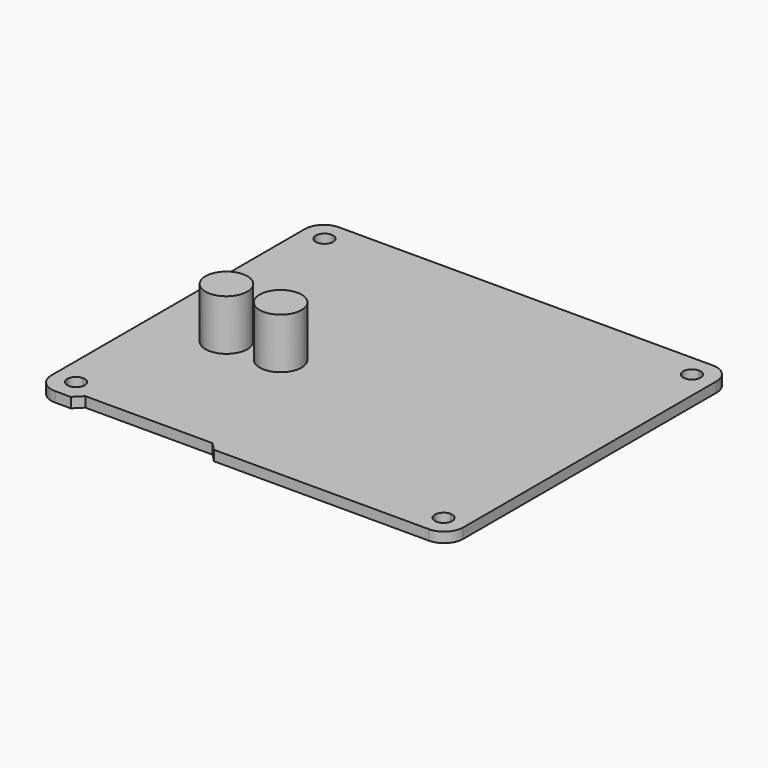
from build123d import *

# Parameters (mm, degrees)
F1_DEPTH = 1.6
F2_R     = 3.3061205596
F2_R_2   = 3.3042251001
F3_DEPTH = 8


# Not quite as in the source:
# - ends of sketch curves that miss each other by under 0.0002 mm in the source are joined


with BuildPart() as f1:
    # F0 (on Top) → F1 (new body)
    with BuildSketch(Plane.XY):
        with BuildLine():
            Line((-30.10027, 26.72715), (-30.10027, -23.27275))
            ThreePointArc((-30.10027, -23.27275), (-29.2216664958, -25.3938864958), (-27.10053, -26.27249))
            Line((-27.10053, -26.27249), (-24.63927, -26.27249))
            Line((-24.63927, -26.27249), (-23.36927, -25.00249))
            Line((-23.36927, -25.00249), (-3.30327, -25.00249))
            Line((-3.30327, -25.00249), (-2.03327, -26.27249))
            Line((-2.03327, -26.27249), (31.89859, -26.27249))
            ThreePointArc((31.89859, -26.27249), (34.020096129, -25.3935121782), (34.9008668601, -23.2727499955))
            Line((34.9008668601, -23.2727499955), (34.90087, 26.72715))
            ThreePointArc((34.90087, 26.72715), (34.0213682803, 28.8491843311), (31.8985900009, 29.7268889246))
            Line((31.8985900009, 29.7268889246), (-27.10053, 29.72689))
            ThreePointArc((-27.10053, 29.72689), (-29.2216664958, 28.8482864958), (-30.10027, 26.72715))
        make_face()
        with BuildLine():
            ThreePointArc((-26.60015, -24.14651), (-27.5718137123, -23.7440337123), (-27.97429, -22.77237))
            ThreePointArc((-27.97429, -22.77237), (-27.5718137123, -21.8007062877), (-26.60015, -21.39823))
            ThreePointArc((-26.60015, -21.39823), (-25.6284862877, -21.8007062877), (-25.22601, -22.77237))
            ThreePointArc((-25.22601, -22.77237), (-25.6284862877, -23.7440337123), (-26.60015, -24.14651))
        make_face(mode=Mode.SUBTRACT)
        with BuildLine():
            ThreePointArc((31.40075, -24.14651), (30.4290862877, -23.7440337123), (30.02661, -22.77237))
            ThreePointArc((30.02661, -22.77237), (30.4290862877, -21.8007062877), (31.40075, -21.39823))
            ThreePointArc((31.40075, -21.39823), (32.3724137123, -21.8007062877), (32.77489, -22.77237))
            ThreePointArc((32.77489, -22.77237), (32.3724137123, -23.7440337123), (31.40075, -24.14651))
        make_face(mode=Mode.SUBTRACT)
        with BuildLine():
            ThreePointArc((-26.60015, 24.8538994131), (-27.5713650107, 25.2559269636), (-27.97429, 26.22677))
            ThreePointArc((-27.97429, 26.22677), (-27.5722630364, 27.1992550107), (-26.60015, 27.6021805869))
            ThreePointArc((-26.60015, 27.6021805869), (-25.6284858727, 27.1997041273), (-25.2260094131, 26.22804))
            ThreePointArc((-25.2260094131, 26.22804), (-25.2260095598, 26.2274049999), (-25.22601, 26.22677))
            ThreePointArc((-25.22601, 26.22677), (-25.6289349893, 25.2559269636), (-26.60015, 24.8538994131))
        make_face(mode=Mode.SUBTRACT)
        with BuildLine():
            ThreePointArc((32.77489, 26.22677), (31.39948, 24.85136), (30.02407, 26.22677))
            ThreePointArc((30.02407, 26.22677), (30.4273673786, 27.1997806471), (31.40075, 27.6021794137))
            ThreePointArc((31.40075, 27.6021794137), (32.3724906471, 27.1988826214), (32.77489, 26.22677))
        make_face(mode=Mode.SUBTRACT)
    extrude(amount=F1_DEPTH)

    # F2 (on face) → F3 (join)
    with BuildSketch(Plane.XY.offset(1.6)):
        with Locations((-18.8942644745, -2.7409724426)):
            Circle(F2_R)
        with Locations((-10.6140207499, -2.4052869994)):
            Circle(F2_R_2)
    extrude(amount=F3_DEPTH)


solid = f1.part
